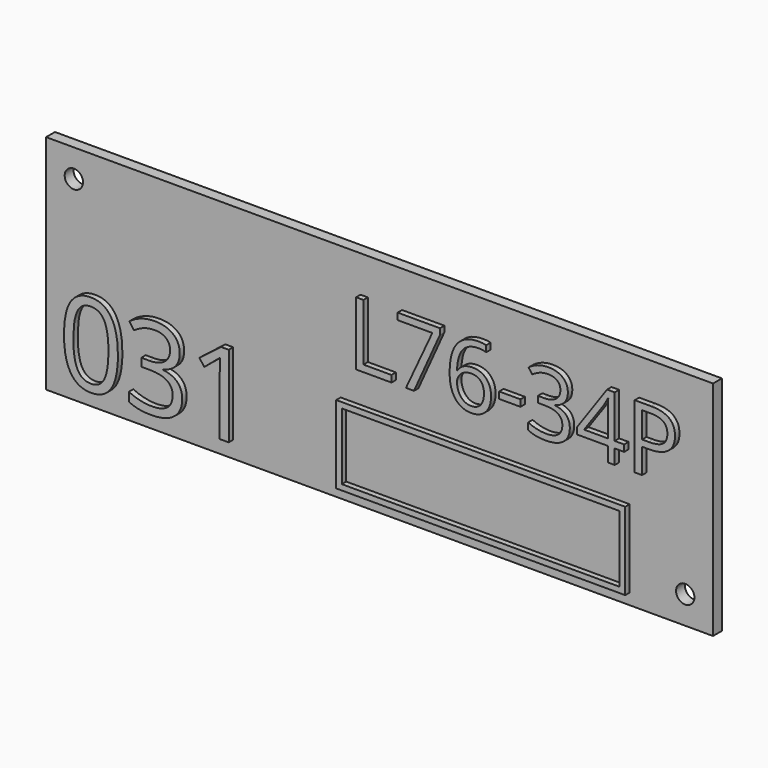
from build123d import *

# Parameters (mm, degrees)
F0_W         = 120
F0_H         = 40
F1_DEPTH     = 2
F3_D         = 3.3
F4_TEXT_SIZE = 16.02871812
F5_DEPTH     = 1
F6_TEXT_SIZE = 20.5478077656
F7_DEPTH     = 1
F8_W         = 52
F8_H         = 14
F8_W_2       = 49.99999962
F8_H_2       = 11.99999962
F9_DEPTH     = 1


# Not quite as in the source:
# - Text() gives the source's letters only with a copy of the font that has no kerning and outlines rounded to 1/6400 em; it was checked with that copy


with BuildPart() as f1:
    # F0 (on Front) → F1 (new body)
    with BuildSketch(Plane.XZ):
        Rectangle(F0_W, F0_H)
    extrude(amount=F1_DEPTH)

    # F3 (through all)
    with Locations(Plane.XZ.offset(2)):
        with Locations((-55, 15), (55, -15)):
            Hole(F3_D / 2)

    # F4 (on face) → F5 (join)
    with BuildSketch(Plane.XZ.offset(2)):
        with Locations((-5, 2)):
            Text('L76-34P', F4_TEXT_SIZE, font='Open Sans', text_align=(TextAlign.LEFT, TextAlign.BOTTOM))
    extrude(amount=F5_DEPTH)

    # F6 (on face) → F7 (join)
    with BuildSketch(Plane.XZ.offset(2)):
        with Locations((-57, -17)):
            Text('031', F6_TEXT_SIZE, font='Open Sans', text_align=(TextAlign.LEFT, TextAlign.BOTTOM))
    extrude(amount=F7_DEPTH)

    # F8 (on face) → F9 (join)
    with BuildSketch(Plane.XZ.offset(2)):
        with Locations((19, -11)):
            Rectangle(F8_W, F8_H)
        with Locations((19, -11)):
            Rectangle(F8_W_2, F8_H_2, mode=Mode.SUBTRACT)
    extrude(amount=F9_DEPTH)


solid = f1.part
